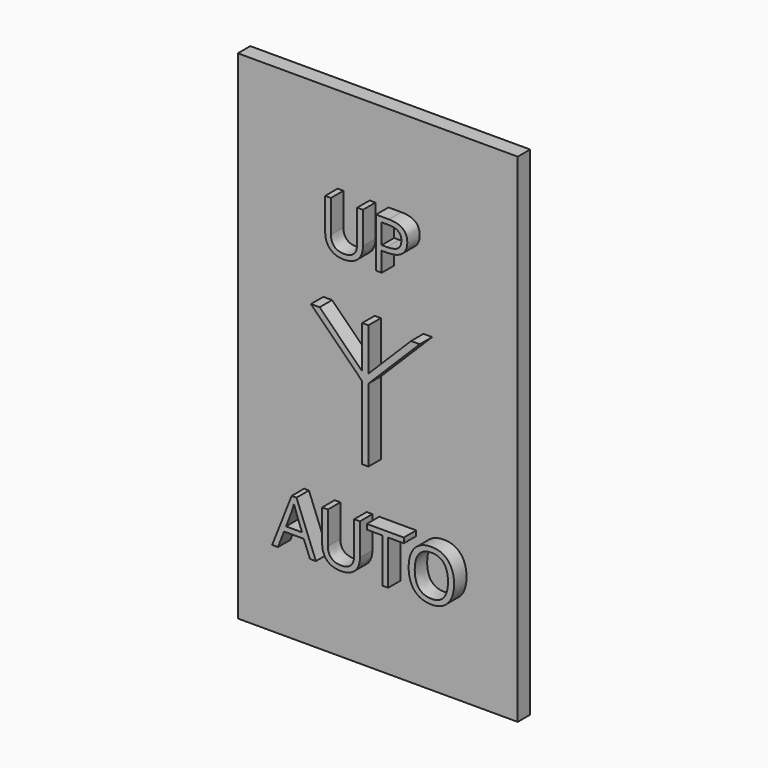
from build123d import *

# Parameters (mm, degrees)
F0_TEXT_SIZE = 4.4444444444
F1_DEPTH     = 1
F3_DEPTH     = 1
F4_W         = 18
F4_H         = 32
F5_DEPTH     = 1


# Not quite as in the source:
# - Text() gives the source's letters only with a copy of the font that has no kerning and outlines rounded to 1/6400 em; it was checked with that copy


with BuildPart() as f1:
    # F0 (on Front) → F1 (new body)
    with BuildSketch(Plane.XZ):
        with Locations((-2.9857638889, 7.25)):
            Text('UP', F0_TEXT_SIZE, font='Open Sans', text_align=(TextAlign.LEFT, TextAlign.BOTTOM))
        with Locations((-5.9927083333, -10.45)):
            Text('AUTO', F0_TEXT_SIZE, font='Open Sans', text_align=(TextAlign.LEFT, TextAlign.BOTTOM))
    extrude(amount=F1_DEPTH)


with BuildPart() as f3:
    # F2 (on Front) → F3 (new body)
    with BuildSketch(Plane.XZ):
        Polygon((0.2, 4), (-0.2, 4), (-0.2, 1.2609940726), (0, 1.0609940726), (0.2, 1.2609940726), align=None)
        Polygon((0, 1.0609940726), (-0.2, 1.2609940726), (-0.2, 0.7009940726), (0, 0.5009940726), (0.2, 0.7009940726), (0.2, 1.2609940726), align=None)
        Polygon((-0.2, 0.7009940726), (-0.2, 1.2609940726), (-2.9390059274, 4), (-3.4990059274, 4), align=None)
        Polygon((2.9390059274, 4), (0.2, 1.2609940726), (0.2, 0.7009940726), (3.4990059274, 4), align=None)
        Polygon((0, 0.5009940726), (-0.2, 0.7009940726), (-0.2, -4), (0.2, -4), (0.2, 0.7009940726), align=None)
    extrude(amount=F3_DEPTH)


with BuildPart() as f5:
    # F4 (on Front) → F5 (new body)
    with BuildSketch(Plane.XZ):
        Rectangle(F4_W, F4_H)
    extrude(amount=-F5_DEPTH)


solid = Compound([f1.part, f3.part, f5.part])
